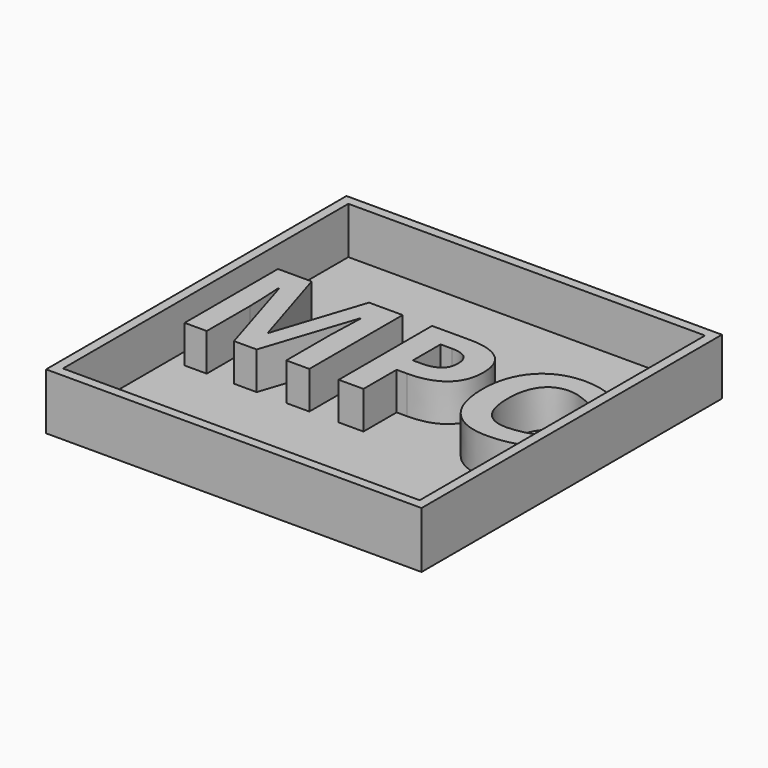
from build123d import *

# Parameters (mm, degrees)
F0_W         = 50.8
F0_H         = 50.8
F1_DEPTH     = 7.62
F2_T         = -1.27
F3_TEXT_SIZE = 22.1124493709
F4_DEPTH     = 5.08


# Not quite as in the source:
# - Text() gives the source's letters only with a copy of the font that has no kerning and outlines rounded to 1/6400 em; it was checked with that copy


with BuildPart() as f1:
    # F0 (on Top) → F1 (new body)
    with BuildSketch(Plane.XY):
        with Locations((-5.9990774184, 16.526710549)):
            Rectangle(F0_W, F0_H)
    extrude(amount=F1_DEPTH)

    # F2
    f2_openings = [f1.faces().sort_by_distance(p)[0] for p in [
        (-5.999077, 16.526711, 7.62),
    ]]
    offset(amount=F2_T, openings=f2_openings)

    # F3 (on face) → F4 (join)
    with BuildSketch(Plane.XY.offset(1.27)):
        with Locations((-30.1290774184, 10.4844596737)):
            Text('MPC', F3_TEXT_SIZE, font='Open Sans', font_style=FontStyle.BOLD, text_align=(TextAlign.LEFT, TextAlign.BOTTOM))
    extrude(amount=F4_DEPTH)


solid = f1.part
